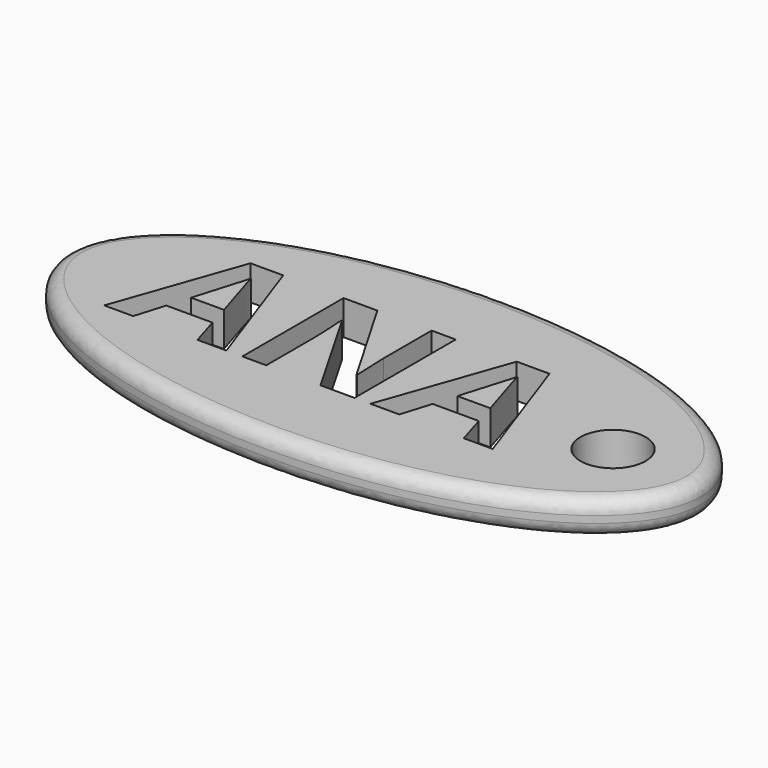
from build123d import *

# Parameters (mm, degrees)
F1_DEPTH     = 3.81
F2_R         = 1.524
F3_R         = 3.6015408846
F3_TEXT_SIZE = 19.5867808846
F4_DEPTH     = 3.8110001


# Not quite as in the source:
# - Text() gives the source's letters only with a copy of the font that has no kerning and outlines rounded to 1/6400 em; it was checked with that copy


with BuildPart() as f1:
    # F0 (on Top) → F1 (new body)
    with BuildSketch(Plane.XY):
        with BuildLine():
            add(Edge.make_bspline(
                [(34.9683985114, 0), (34.9683985114, 28.4775254861), (-17.4841992557, 14.238762743), (-69.9367970228, 0), (-17.4841992557, -14.238762743), (34.9683985114, -28.4775254861), (34.9683985114, 0)],
                knots=[0, 0, 0, 2.0943951024, 2.0943951024, 4.1887902048, 4.1887902048, 6.2831853072, 6.2831853072, 6.2831853072], degree=2, weights=[1, 0.5, 1, 0.5, 1, 0.5, 1]))
        make_face()
    extrude(amount=F1_DEPTH)

    # F2
    f2_edges = [f1.edges().sort_by_distance(p)[0] for p in [
        (-34.968399, 9e-06, 3.81),
        (-34.968399, 9e-06, 0),
    ]]
    fillet(f2_edges, radius=F2_R)

    # F3 (on face) → F4 (cut, through all)
    with BuildSketch(Plane.XY.offset(3.81)):
        with Locations((25.3226421773, 0)):
            Circle(F3_R)
        with Locations((-25.7586147636, -6.4756297506)):
            Text('ANA', F3_TEXT_SIZE, font='Open Sans', font_style=FontStyle.BOLD, text_align=(TextAlign.LEFT, TextAlign.BOTTOM))
    extrude(amount=-F4_DEPTH, mode=Mode.SUBTRACT)


solid = f1.part
